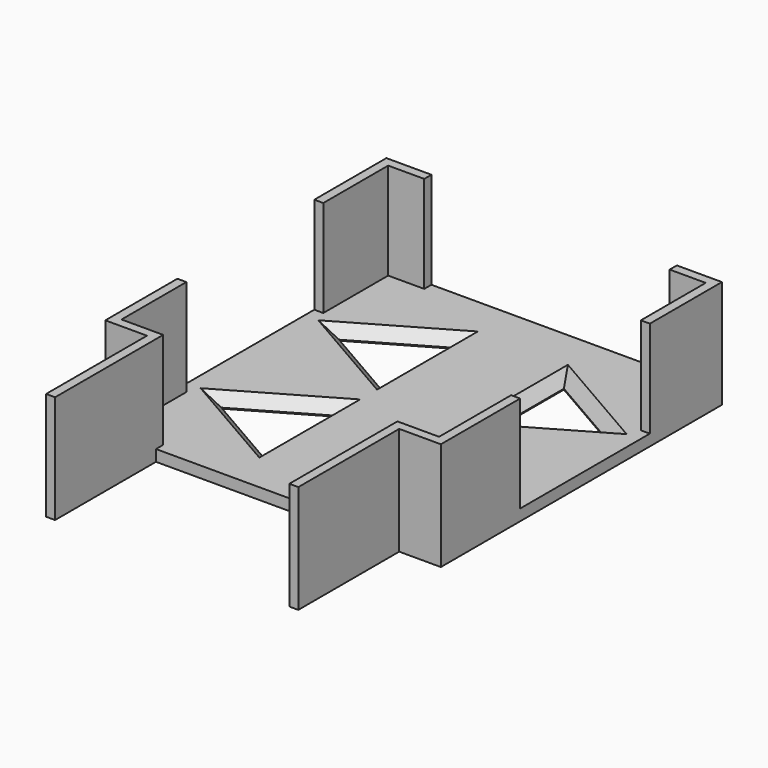
from build123d import *

# Parameters (mm, degrees)
F0_W     = 26
F0_H     = 2
F0_W_2   = 27.25
F0_W_3   = 2
F0_H_2   = 36
F0_H_3   = 38
F1_DEPTH = 2.5
F2_SIZE  = 2.3
F0_H_4   = 28
F3_DEPTH = 24


with BuildPart() as f1:
    # F0 (on Top) → F1 (new body)
    with BuildSketch(Plane.XY):
        Polygon((0, 37), (0, -37), (26, -37), (35.25, -37), (35.25, -17), (35.25, 19), (35.25, 37), (27.25, 37), align=None)
        Polygon((12.302681016, -26.3321439177), (12.302681016, -6.3321439177), (29.6231890917, -16.3321439177), align=None, mode=Mode.SUBTRACT)
        Polygon((12.302681016, 26.3321439177), (29.6231890917, 16.3321439177), (12.302681016, 6.3321439177), align=None, mode=Mode.SUBTRACT)
        Polygon((-35.25, 19), (-35.25, -19), (-35.25, -37), (-26, -37), (0, -37), (0, 37), (-27.25, 37), (-35.25, 37), align=None)
        Polygon((-12.302681016, -26.3321439177), (-29.6231890917, -16.3321439177), (-12.302681016, -6.3321439177), align=None, mode=Mode.SUBTRACT)
        Polygon((-12.302681016, 26.3321439177), (-12.302681016, 6.3321439177), (-29.6231890917, 16.3321439177), align=None, mode=Mode.SUBTRACT)
        with Locations((-13, -38)):
            Rectangle(F0_W, F0_H)
        with Locations((13, -38)):
            Rectangle(F0_W, F0_H)
        with Locations((-13.625, 38)):
            Rectangle(F0_W_2, F0_H)
        with Locations((13.625, 38)):
            Rectangle(F0_W_2, F0_H)
        with Locations((36.25, 1)):
            Rectangle(F0_W_3, F0_H_2)
        with Locations((-36.25, 0)):
            Rectangle(F0_W_3, F0_H_3)
    extrude(amount=F1_DEPTH)

    # F2
    f2_edges = [f1.edges().sort_by_distance(p)[0] for p in [
        (-20.962935, -11.332144, 2.5),
        (-20.962935, -21.332144, 2.5),
        (-12.302681, -16.332144, 2.5),
        (20.962935, -11.332144, 2.5),
        (12.302681, -16.332144, 2.5),
        (20.962935, -21.332144, 2.5),
        (20.962935, 21.332144, 2.5),
        (12.302681, 16.332144, 2.5),
        (20.962935, 11.332144, 2.5),
        (-20.962935, 21.332144, 2.5),
        (-20.962935, 11.332144, 2.5),
        (-12.302681, 16.332144, 2.5),
    ]]
    chamfer(f2_edges, length=F2_SIZE)

    # F0 (on Top) → F3 (join)
    with BuildSketch(Plane.XY):
        Polygon((-37.25, 39), (-37.25, 19), (-35.25, 19), (-35.25, 37), (-27.25, 37), (-27.25, 39), align=None)
        Polygon((27.25, 39), (27.25, 37), (35.25, 37), (35.25, 19), (37.25, 19), (37.25, 39), align=None)
        Polygon((26, -37), (26, -39), (28, -39), (37.25, -39), (37.25, -17), (35.25, -17), (35.25, -37), align=None)
        Polygon((-37.25, -19), (-37.25, -39), (-28, -39), (-26, -39), (-26, -37), (-35.25, -37), (-35.25, -19), align=None)
        with Locations((27, -53)):
            Rectangle(F0_W_3, F0_H_4)
        with Locations((-27, -53)):
            Rectangle(F0_W_3, F0_H_4)
    extrude(amount=F3_DEPTH)


solid = f1.part
